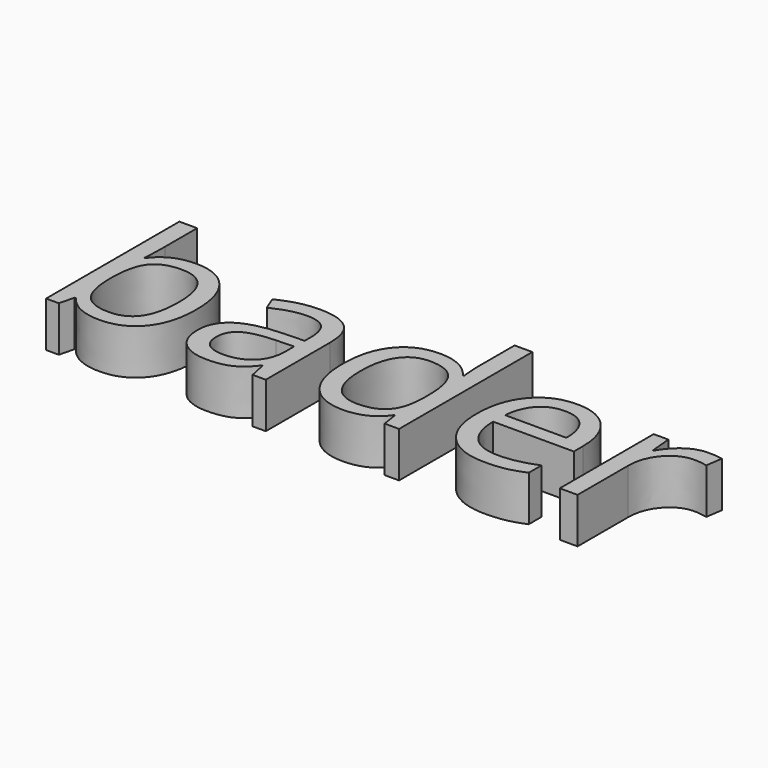
from build123d import *

# Parameters (mm, degrees)
F0_TEXT_SIZE = 24.1650087345
F1_DEPTH     = 5


# Not quite as in the source:
# - Text() gives the source's letters only with a copy of the font that has no kerning and outlines rounded to 1/6400 em; it was checked with that copy


with BuildPart() as f1:
    # F0 (on Top) → F1 (new body)
    with BuildSketch(Plane.XY):
        with Locations((0, 0)):
            Text('bader', F0_TEXT_SIZE, font='Open Sans', text_align=(TextAlign.LEFT, TextAlign.BOTTOM))
    extrude(amount=F1_DEPTH)


solid = f1.part
